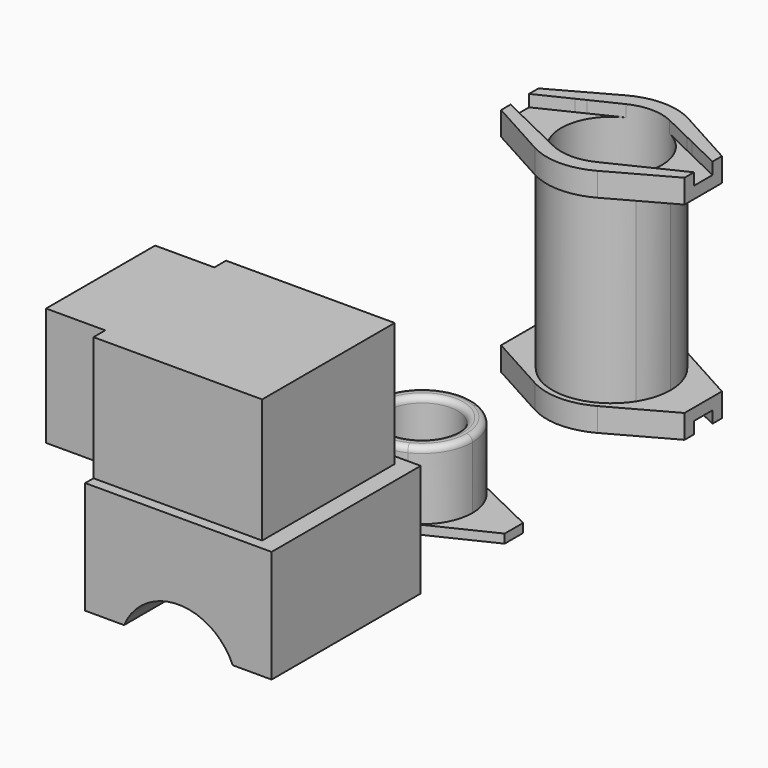
from build123d import *

# Parameters (mm, degrees)
F1_DEPTH  = 1.905
F0_R      = 7.5565
F2_DEPTH  = 16.51
F3_R      = 1.27
F5_DEPTH  = 49.53
F6_DEPTH  = 44.45
F7_DEPTH  = 5.08
F8_DEPTH  = 49.53
F9_DEPTH  = 46.99
F10_DEPTH = 44.45
F11_DEPTH = 5.08
F12_DEPTH = 2.54
F13_DEPTH = 49.53
F15_DEPTH = 24.13
F16_DEPTH = 50.8
F14_W     = 12.7
F14_H     = 29.2608
F17_DEPTH = 50.8
F18_DEPTH = 15.875
F19_DEPTH = 25.4
F21_DEPTH = 5.08
F22_DEPTH = 40.005


# Not quite as in the source:
# - after a boolean that leaves OpenCascade's solid faulty, fix() repairs it


with BuildPart() as f1:
    # F0 (on Top) → F1 (new body)
    with BuildSketch(Plane.XY):
        with BuildLine():
            ThreePointArc((-4.6970553339, -9.7195522628), (-10.795, -1.92e-08), (-4.6970553686, 9.7195522461))
            Line((-4.6970553686, 9.7195522461), (-19.685, 2.4765))
            Line((-19.685, 2.4765), (-19.685, -2.4765))
            Line((-19.685, -2.4765), (-4.6970553339, -9.7195522628))
        make_face()
    extrude(amount=F1_DEPTH)



with BuildPart() as f1b:
    # F0 (on Top) → F1, piece 2 (new body)
    with BuildSketch(Plane.XY):
        with BuildLine():
            ThreePointArc((4.6970552092, 9.7195523231), (9.1443079559, 5.7370425315), (10.795, 0))
            ThreePointArc((10.795, 0), (9.1443079608, -5.7370425236), (4.697055226, -9.719552315))
            Line((4.697055226, -9.719552315), (19.685, -2.4765))
            Line((19.685, -2.4765), (19.685, 2.4765))
            Line((19.685, 2.4765), (4.6970552092, 9.7195523231))
        make_face()
    extrude(amount=F1_DEPTH)


with BuildPart() as f1_1:
    add(f1.part)

    add(f1b.part)  # F2 merges F1b
    # F0 (on Top) → F2 (join)
    with BuildSketch(Plane.XY):
        with BuildLine():
            ThreePointArc((4.697055226, -9.719552315), (9.1443079608, -5.7370425236), (10.795, 0))
            ThreePointArc((10.795, 0), (9.1443079559, 5.7370425315), (4.6970552092, 9.7195523231))
            ThreePointArc((4.6970552092, 9.7195523231), (-8.85e-08, 10.795), (-4.6970553686, 9.7195522461))
            ThreePointArc((-4.6970553686, 9.7195522461), (-10.795, -1.92e-08), (-4.6970553339, -9.7195522628))
            ThreePointArc((-4.6970553339, -9.7195522628), (-5.99e-08, -10.795), (4.697055226, -9.719552315))
        make_face()
        Circle(F0_R, mode=Mode.SUBTRACT)
    extrude(amount=F2_DEPTH)

    # F3
    f3_edges = [f1_1.edges().sort_by_distance(p)[0] for p in [
        (-7.5565, 0, 16.51),
        (-4.697055, -9.719552, 16.51),
    ]]
    fillet(f3_edges, radius=F3_R)


with BuildPart() as f5:
    # F4 (on Top) → F5 (new body)
    with BuildSketch(Plane.XY):
        with BuildLine():
            ThreePointArc((-6.7218508036, 38.6259512066), (-10.1522301266, 41.2961604755), (-12.5905662524, 44.8950543022))
            Line((-12.5905662524, 44.8950543022), (-19.685, 48.3235))
            Line((-19.685, 48.3235), (-19.685, 45.7835))
            Line((-19.685, 45.7835), (-6.7218508036, 38.6259512066))
        make_face()
        with BuildLine():
            Line((19.685, 48.3235), (12.5905662524, 44.8950543022))
            ThreePointArc((12.5905662524, 44.8950543022), (10.1522300664, 41.2961604112), (6.7218506494, 38.6259511215))
            Line((6.7218506494, 38.6259511215), (19.685, 45.7835))
            Line((19.685, 45.7835), (19.685, 48.3235))
        make_face()
        with BuildLine():
            ThreePointArc((6.7218505572, 62.9740489294), (10.1522300304, 60.3038396273), (12.5905662524, 56.7049456978))
            Line((12.5905662524, 56.7049456978), (19.685, 53.2765))
            Line((19.685, 53.2765), (19.685, 55.8165))
            Line((19.685, 55.8165), (6.7218505572, 62.9740489294))
        make_face()
        with BuildLine():
            Line((-19.685, 53.2765), (-12.5905662524, 56.7049456978))
            ThreePointArc((-12.5905662524, 56.7049456978), (-10.1522299741, 60.3038396874), (-6.721850413, 62.9740490091))
            Line((-6.721850413, 62.9740490091), (-19.685, 55.8165))
            Line((-19.685, 55.8165), (-19.685, 53.2765))
        make_face()
        with BuildLine():
            ThreePointArc((-12.5905662524, 44.8950543022), (-13.9065, 50.8), (-12.5905662524, 56.7049456978))
            Line((-12.5905662524, 56.7049456978), (-19.685, 53.2765))
            Line((-19.685, 53.2765), (-19.685, 48.3235))
            Line((-19.685, 48.3235), (-12.5905662524, 44.8950543022))
        make_face()
        with BuildLine():
            Line((19.685, 53.2765), (12.5905662524, 56.7049456978))
            ThreePointArc((12.5905662524, 56.7049456978), (13.5735303411, 53.8248993918), (13.9065, 50.8))
            ThreePointArc((13.9065, 50.8), (13.5735303411, 47.7751006082), (12.5905662524, 44.8950543022))
            Line((12.5905662524, 44.8950543022), (19.685, 48.3235))
            Line((19.685, 48.3235), (19.685, 53.2765))
        make_face()
        with BuildLine():
            ThreePointArc((-10.7206935622, 43.9914223552), (-12.7, 50.8), (-10.7206935622, 57.6085776448))
            Line((-10.7206935622, 57.6085776448), (-12.5905662524, 56.7049456978))
            ThreePointArc((-12.5905662524, 56.7049456978), (-13.9065, 50.8), (-12.5905662524, 44.8950543022))
            Line((-12.5905662524, 44.8950543022), (-10.7206935622, 43.9914223552))
        make_face()
        with BuildLine():
            ThreePointArc((-10.7206935622, 57.6085776448), (0, 63.5), (10.7206935622, 57.6085776448))
            Line((10.7206935622, 57.6085776448), (12.5905662524, 56.7049456978))
            ThreePointArc((12.5905662524, 56.7049456978), (10.1522300304, 60.3038396273), (6.7218505572, 62.9740489294))
            ThreePointArc((6.7218505572, 62.9740489294), (8.24e-08, 64.7065), (-6.721850413, 62.9740490091))
            ThreePointArc((-6.721850413, 62.9740490091), (-10.1522299741, 60.3038396874), (-12.5905662524, 56.7049456978))
            Line((-12.5905662524, 56.7049456978), (-10.7206935622, 57.6085776448))
        make_face()
        with BuildLine():
            ThreePointArc((-4.6970550571, 41.0804476034), (-10.795, 50.7999998253), (-4.6970553717, 60.5195522446))
            Line((-4.6970553717, 60.5195522446), (-10.7206935622, 57.6085776448))
            ThreePointArc((-10.7206935622, 57.6085776448), (-12.7, 50.8), (-10.7206935622, 43.9914223552))
            Line((-10.7206935622, 43.9914223552), (-4.6970550571, 41.0804476034))
        make_face()
        with BuildLine():
            Line((0, 62.7894443677), (4.697055398, 60.5195522319))
            Line((4.697055398, 60.5195522319), (10.7206935622, 57.6085776448))
            ThreePointArc((10.7206935622, 57.6085776448), (0, 63.5), (-10.7206935622, 57.6085776448))
            Line((-10.7206935622, 57.6085776448), (-4.6970553717, 60.5195522446))
            Line((-4.6970553717, 60.5195522446), (0, 62.7894443677))
        make_face()
        with BuildLine():
            ThreePointArc((-4.6970553717, 60.5195522446), (1.46e-08, 61.595), (4.697055398, 60.5195522319))
            Line((4.697055398, 60.5195522319), (0, 62.7894443677))
            Line((0, 62.7894443677), (-4.6970553717, 60.5195522446))
        make_face()
        with BuildLine():
            ThreePointArc((4.6970554112, 41.0804477745), (9.1443080155, 45.0629575635), (10.795, 50.8))
            ThreePointArc((10.795, 50.8), (9.1443080116, 56.5370424427), (4.697055398, 60.5195522319))
            ThreePointArc((4.697055398, 60.5195522319), (1.46e-08, 61.595), (-4.6970553717, 60.5195522446))
            ThreePointArc((-4.6970553717, 60.5195522446), (-10.795, 50.7999998253), (-4.6970550571, 41.0804476034))
            ThreePointArc((-4.6970550571, 41.0804476034), (1.966e-07, 40.005), (4.6970554112, 41.0804477745))
        make_face()
        with BuildLine():
            Line((0, 38.8105556323), (4.6970554112, 41.0804477745))
            ThreePointArc((4.6970554112, 41.0804477745), (1.966e-07, 40.005), (-4.6970550571, 41.0804476034))
            Line((-4.6970550571, 41.0804476034), (0, 38.8105556323))
        make_face()
        with BuildLine():
            Line((10.7206935622, 43.9914223552), (4.6970554112, 41.0804477745))
            Line((4.6970554112, 41.0804477745), (0, 38.8105556323))
            Line((0, 38.8105556323), (-4.6970550571, 41.0804476034))
            Line((-4.6970550571, 41.0804476034), (-10.7206935622, 43.9914223552))
            ThreePointArc((-10.7206935622, 43.9914223552), (0, 38.1), (10.7206935622, 43.9914223552))
        make_face()
        with BuildLine():
            Line((12.5905662524, 44.8950543022), (10.7206935622, 43.9914223552))
            ThreePointArc((10.7206935622, 43.9914223552), (0, 38.1), (-10.7206935622, 43.9914223552))
            Line((-10.7206935622, 43.9914223552), (-12.5905662524, 44.8950543022))
            ThreePointArc((-12.5905662524, 44.8950543022), (-10.1522301266, 41.2961604755), (-6.7218508036, 38.6259512066))
            ThreePointArc((-6.7218508036, 38.6259512066), (-8.81e-08, 36.8935), (6.7218506494, 38.6259511215))
            ThreePointArc((6.7218506494, 38.6259511215), (10.1522300664, 41.2961604112), (12.5905662524, 44.8950543022))
        make_face()
        with BuildLine():
            ThreePointArc((4.697055398, 60.5195522319), (9.1443080116, 56.5370424427), (10.795, 50.8))
            ThreePointArc((10.795, 50.8), (9.1443080155, 45.0629575635), (4.6970554112, 41.0804477745))
            Line((4.6970554112, 41.0804477745), (10.7206935622, 43.9914223552))
            ThreePointArc((10.7206935622, 43.9914223552), (12.1951385445, 47.2547784442), (12.7, 50.8))
            ThreePointArc((12.7, 50.8), (12.1951385445, 54.3452215558), (10.7206935622, 57.6085776448))
            Line((10.7206935622, 57.6085776448), (4.697055398, 60.5195522319))
        make_face()
        with BuildLine():
            Line((12.5905662524, 56.7049456978), (10.7206935622, 57.6085776448))
            ThreePointArc((10.7206935622, 57.6085776448), (12.1951385445, 54.3452215558), (12.7, 50.8))
            ThreePointArc((12.7, 50.8), (12.1951385445, 47.2547784442), (10.7206935622, 43.9914223552))
            Line((10.7206935622, 43.9914223552), (12.5905662524, 44.8950543022))
            ThreePointArc((12.5905662524, 44.8950543022), (13.5735303411, 47.7751006082), (13.9065, 50.8))
            ThreePointArc((13.9065, 50.8), (13.5735303411, 53.8248993918), (12.5905662524, 56.7049456978))
        make_face()
    extrude(amount=F5_DEPTH)

    # F4 (on Top) → F6 (cut)
    with BuildSketch(Plane.XY):
        with BuildLine():
            ThreePointArc((-6.7218508036, 38.6259512066), (-10.1522301266, 41.2961604755), (-12.5905662524, 44.8950543022))
            Line((-12.5905662524, 44.8950543022), (-19.685, 48.3235))
            Line((-19.685, 48.3235), (-19.685, 45.7835))
            Line((-19.685, 45.7835), (-6.7218508036, 38.6259512066))
        make_face()
        with BuildLine():
            ThreePointArc((-12.5905662524, 44.8950543022), (-13.9065, 50.8), (-12.5905662524, 56.7049456978))
            Line((-12.5905662524, 56.7049456978), (-19.685, 53.2765))
            Line((-19.685, 53.2765), (-19.685, 48.3235))
            Line((-19.685, 48.3235), (-12.5905662524, 44.8950543022))
        make_face()
        with BuildLine():
            Line((-19.685, 53.2765), (-12.5905662524, 56.7049456978))
            ThreePointArc((-12.5905662524, 56.7049456978), (-10.1522299741, 60.3038396874), (-6.721850413, 62.9740490091))
            Line((-6.721850413, 62.9740490091), (-19.685, 55.8165))
            Line((-19.685, 55.8165), (-19.685, 53.2765))
        make_face()
        with BuildLine():
            ThreePointArc((6.7218505572, 62.9740489294), (10.1522300304, 60.3038396273), (12.5905662524, 56.7049456978))
            Line((12.5905662524, 56.7049456978), (19.685, 53.2765))
            Line((19.685, 53.2765), (19.685, 55.8165))
            Line((19.685, 55.8165), (6.7218505572, 62.9740489294))
        make_face()
        with BuildLine():
            Line((19.685, 53.2765), (12.5905662524, 56.7049456978))
            ThreePointArc((12.5905662524, 56.7049456978), (13.5735303411, 53.8248993918), (13.9065, 50.8))
            ThreePointArc((13.9065, 50.8), (13.5735303411, 47.7751006082), (12.5905662524, 44.8950543022))
            Line((12.5905662524, 44.8950543022), (19.685, 48.3235))
            Line((19.685, 48.3235), (19.685, 53.2765))
        make_face()
        with BuildLine():
            Line((19.685, 48.3235), (12.5905662524, 44.8950543022))
            ThreePointArc((12.5905662524, 44.8950543022), (10.1522300664, 41.2961604112), (6.7218506494, 38.6259511215))
            Line((6.7218506494, 38.6259511215), (19.685, 45.7835))
            Line((19.685, 45.7835), (19.685, 48.3235))
        make_face()
        with BuildLine():
            Line((12.5905662524, 44.8950543022), (10.7206935622, 43.9914223552))
            ThreePointArc((10.7206935622, 43.9914223552), (0, 38.1), (-10.7206935622, 43.9914223552))
            Line((-10.7206935622, 43.9914223552), (-12.5905662524, 44.8950543022))
            ThreePointArc((-12.5905662524, 44.8950543022), (-10.1522301266, 41.2961604755), (-6.7218508036, 38.6259512066))
            ThreePointArc((-6.7218508036, 38.6259512066), (-8.81e-08, 36.8935), (6.7218506494, 38.6259511215))
            ThreePointArc((6.7218506494, 38.6259511215), (10.1522300664, 41.2961604112), (12.5905662524, 44.8950543022))
        make_face()
        with BuildLine():
            ThreePointArc((-10.7206935622, 57.6085776448), (0, 63.5), (10.7206935622, 57.6085776448))
            Line((10.7206935622, 57.6085776448), (12.5905662524, 56.7049456978))
            ThreePointArc((12.5905662524, 56.7049456978), (10.1522300304, 60.3038396273), (6.7218505572, 62.9740489294))
            ThreePointArc((6.7218505572, 62.9740489294), (8.24e-08, 64.7065), (-6.721850413, 62.9740490091))
            ThreePointArc((-6.721850413, 62.9740490091), (-10.1522299741, 60.3038396874), (-12.5905662524, 56.7049456978))
            Line((-12.5905662524, 56.7049456978), (-10.7206935622, 57.6085776448))
        make_face()
        with BuildLine():
            Line((12.5905662524, 56.7049456978), (10.7206935622, 57.6085776448))
            ThreePointArc((10.7206935622, 57.6085776448), (12.1951385445, 54.3452215558), (12.7, 50.8))
            ThreePointArc((12.7, 50.8), (12.1951385445, 47.2547784442), (10.7206935622, 43.9914223552))
            Line((10.7206935622, 43.9914223552), (12.5905662524, 44.8950543022))
            ThreePointArc((12.5905662524, 44.8950543022), (13.5735303411, 47.7751006082), (13.9065, 50.8))
            ThreePointArc((13.9065, 50.8), (13.5735303411, 53.8248993918), (12.5905662524, 56.7049456978))
        make_face()
        with BuildLine():
            ThreePointArc((-10.7206935622, 43.9914223552), (-12.7, 50.8), (-10.7206935622, 57.6085776448))
            Line((-10.7206935622, 57.6085776448), (-12.5905662524, 56.7049456978))
            ThreePointArc((-12.5905662524, 56.7049456978), (-13.9065, 50.8), (-12.5905662524, 44.8950543022))
            Line((-12.5905662524, 44.8950543022), (-10.7206935622, 43.9914223552))
        make_face()
    extrude(amount=F6_DEPTH, mode=Mode.SUBTRACT)

    # F4 (on Top) → F7 (join)
    with BuildSketch(Plane.XY):
        with BuildLine():
            ThreePointArc((-6.7218508036, 38.6259512066), (-10.1522301266, 41.2961604755), (-12.5905662524, 44.8950543022))
            Line((-12.5905662524, 44.8950543022), (-19.685, 48.3235))
            Line((-19.685, 48.3235), (-19.685, 45.7835))
            Line((-19.685, 45.7835), (-6.7218508036, 38.6259512066))
        make_face()
        with BuildLine():
            Line((12.5905662524, 44.8950543022), (10.7206935622, 43.9914223552))
            ThreePointArc((10.7206935622, 43.9914223552), (0, 38.1), (-10.7206935622, 43.9914223552))
            Line((-10.7206935622, 43.9914223552), (-12.5905662524, 44.8950543022))
            ThreePointArc((-12.5905662524, 44.8950543022), (-10.1522301266, 41.2961604755), (-6.7218508036, 38.6259512066))
            ThreePointArc((-6.7218508036, 38.6259512066), (-8.81e-08, 36.8935), (6.7218506494, 38.6259511215))
            ThreePointArc((6.7218506494, 38.6259511215), (10.1522300664, 41.2961604112), (12.5905662524, 44.8950543022))
        make_face()
        with BuildLine():
            Line((10.7206935622, 43.9914223552), (4.6970554112, 41.0804477745))
            Line((4.6970554112, 41.0804477745), (0, 38.8105556323))
            Line((0, 38.8105556323), (-4.6970550571, 41.0804476034))
            Line((-4.6970550571, 41.0804476034), (-10.7206935622, 43.9914223552))
            ThreePointArc((-10.7206935622, 43.9914223552), (0, 38.1), (10.7206935622, 43.9914223552))
        make_face()
        with BuildLine():
            ThreePointArc((-4.6970550571, 41.0804476034), (-10.795, 50.7999998253), (-4.6970553717, 60.5195522446))
            Line((-4.6970553717, 60.5195522446), (-10.7206935622, 57.6085776448))
            ThreePointArc((-10.7206935622, 57.6085776448), (-12.7, 50.8), (-10.7206935622, 43.9914223552))
            Line((-10.7206935622, 43.9914223552), (-4.6970550571, 41.0804476034))
        make_face()
        with BuildLine():
            ThreePointArc((-10.7206935622, 43.9914223552), (-12.7, 50.8), (-10.7206935622, 57.6085776448))
            Line((-10.7206935622, 57.6085776448), (-12.5905662524, 56.7049456978))
            ThreePointArc((-12.5905662524, 56.7049456978), (-13.9065, 50.8), (-12.5905662524, 44.8950543022))
            Line((-12.5905662524, 44.8950543022), (-10.7206935622, 43.9914223552))
        make_face()
        with BuildLine():
            ThreePointArc((-12.5905662524, 44.8950543022), (-13.9065, 50.8), (-12.5905662524, 56.7049456978))
            Line((-12.5905662524, 56.7049456978), (-19.685, 53.2765))
            Line((-19.685, 53.2765), (-19.685, 48.3235))
            Line((-19.685, 48.3235), (-12.5905662524, 44.8950543022))
        make_face()
        with BuildLine():
            Line((-19.685, 53.2765), (-12.5905662524, 56.7049456978))
            ThreePointArc((-12.5905662524, 56.7049456978), (-10.1522299741, 60.3038396874), (-6.721850413, 62.9740490091))
            Line((-6.721850413, 62.9740490091), (-19.685, 55.8165))
            Line((-19.685, 55.8165), (-19.685, 53.2765))
        make_face()
        with BuildLine():
            Line((0, 62.7894443677), (4.697055398, 60.5195522319))
            Line((4.697055398, 60.5195522319), (10.7206935622, 57.6085776448))
            ThreePointArc((10.7206935622, 57.6085776448), (0, 63.5), (-10.7206935622, 57.6085776448))
            Line((-10.7206935622, 57.6085776448), (-4.6970553717, 60.5195522446))
            Line((-4.6970553717, 60.5195522446), (0, 62.7894443677))
        make_face()
        with BuildLine():
            ThreePointArc((-10.7206935622, 57.6085776448), (0, 63.5), (10.7206935622, 57.6085776448))
            Line((10.7206935622, 57.6085776448), (12.5905662524, 56.7049456978))
            ThreePointArc((12.5905662524, 56.7049456978), (10.1522300304, 60.3038396273), (6.7218505572, 62.9740489294))
            ThreePointArc((6.7218505572, 62.9740489294), (8.24e-08, 64.7065), (-6.721850413, 62.9740490091))
            ThreePointArc((-6.721850413, 62.9740490091), (-10.1522299741, 60.3038396874), (-12.5905662524, 56.7049456978))
            Line((-12.5905662524, 56.7049456978), (-10.7206935622, 57.6085776448))
        make_face()
        with BuildLine():
            ThreePointArc((-4.6970553717, 60.5195522446), (1.46e-08, 61.595), (4.697055398, 60.5195522319))
            Line((4.697055398, 60.5195522319), (0, 62.7894443677))
            Line((0, 62.7894443677), (-4.6970553717, 60.5195522446))
        make_face()
        with BuildLine():
            ThreePointArc((4.6970554112, 41.0804477745), (9.1443080155, 45.0629575635), (10.795, 50.8))
            ThreePointArc((10.795, 50.8), (9.1443080116, 56.5370424427), (4.697055398, 60.5195522319))
            ThreePointArc((4.697055398, 60.5195522319), (1.46e-08, 61.595), (-4.6970553717, 60.5195522446))
            ThreePointArc((-4.6970553717, 60.5195522446), (-10.795, 50.7999998253), (-4.6970550571, 41.0804476034))
            ThreePointArc((-4.6970550571, 41.0804476034), (1.966e-07, 40.005), (4.6970554112, 41.0804477745))
        make_face()
        with BuildLine():
            ThreePointArc((4.697055398, 60.5195522319), (9.1443080116, 56.5370424427), (10.795, 50.8))
            ThreePointArc((10.795, 50.8), (9.1443080155, 45.0629575635), (4.6970554112, 41.0804477745))
            Line((4.6970554112, 41.0804477745), (10.7206935622, 43.9914223552))
            ThreePointArc((10.7206935622, 43.9914223552), (12.1951385445, 47.2547784442), (12.7, 50.8))
            ThreePointArc((12.7, 50.8), (12.1951385445, 54.3452215558), (10.7206935622, 57.6085776448))
            Line((10.7206935622, 57.6085776448), (4.697055398, 60.5195522319))
        make_face()
        with BuildLine():
            Line((12.5905662524, 56.7049456978), (10.7206935622, 57.6085776448))
            ThreePointArc((10.7206935622, 57.6085776448), (12.1951385445, 54.3452215558), (12.7, 50.8))
            ThreePointArc((12.7, 50.8), (12.1951385445, 47.2547784442), (10.7206935622, 43.9914223552))
            Line((10.7206935622, 43.9914223552), (12.5905662524, 44.8950543022))
            ThreePointArc((12.5905662524, 44.8950543022), (13.5735303411, 47.7751006082), (13.9065, 50.8))
            ThreePointArc((13.9065, 50.8), (13.5735303411, 53.8248993918), (12.5905662524, 56.7049456978))
        make_face()
        with BuildLine():
            Line((19.685, 53.2765), (12.5905662524, 56.7049456978))
            ThreePointArc((12.5905662524, 56.7049456978), (13.5735303411, 53.8248993918), (13.9065, 50.8))
            ThreePointArc((13.9065, 50.8), (13.5735303411, 47.7751006082), (12.5905662524, 44.8950543022))
            Line((12.5905662524, 44.8950543022), (19.685, 48.3235))
            Line((19.685, 48.3235), (19.685, 53.2765))
        make_face()
        with BuildLine():
            ThreePointArc((6.7218505572, 62.9740489294), (10.1522300304, 60.3038396273), (12.5905662524, 56.7049456978))
            Line((12.5905662524, 56.7049456978), (19.685, 53.2765))
            Line((19.685, 53.2765), (19.685, 55.8165))
            Line((19.685, 55.8165), (6.7218505572, 62.9740489294))
        make_face()
        with BuildLine():
            Line((19.685, 48.3235), (12.5905662524, 44.8950543022))
            ThreePointArc((12.5905662524, 44.8950543022), (10.1522300664, 41.2961604112), (6.7218506494, 38.6259511215))
            Line((6.7218506494, 38.6259511215), (19.685, 45.7835))
            Line((19.685, 45.7835), (19.685, 48.3235))
        make_face()
        with BuildLine():
            Line((0, 38.8105556323), (4.6970554112, 41.0804477745))
            ThreePointArc((4.6970554112, 41.0804477745), (1.966e-07, 40.005), (-4.6970550571, 41.0804476034))
            Line((-4.6970550571, 41.0804476034), (0, 38.8105556323))
        make_face()
    extrude(amount=F7_DEPTH)

    # F4 (on Top) → F8 (cut)
    with BuildSketch(Plane.XY):
        with BuildLine():
            ThreePointArc((-12.5905662524, 44.8950543022), (-13.9065, 50.8), (-12.5905662524, 56.7049456978))
            Line((-12.5905662524, 56.7049456978), (-19.685, 53.2765))
            Line((-19.685, 53.2765), (-19.685, 48.3235))
            Line((-19.685, 48.3235), (-12.5905662524, 44.8950543022))
        make_face()
        with BuildLine():
            ThreePointArc((-10.7206935622, 43.9914223552), (-12.7, 50.8), (-10.7206935622, 57.6085776448))
            Line((-10.7206935622, 57.6085776448), (-12.5905662524, 56.7049456978))
            ThreePointArc((-12.5905662524, 56.7049456978), (-13.9065, 50.8), (-12.5905662524, 44.8950543022))
            Line((-12.5905662524, 44.8950543022), (-10.7206935622, 43.9914223552))
        make_face()
        with BuildLine():
            ThreePointArc((-4.6970550571, 41.0804476034), (-10.795, 50.7999998253), (-4.6970553717, 60.5195522446))
            Line((-4.6970553717, 60.5195522446), (-10.7206935622, 57.6085776448))
            ThreePointArc((-10.7206935622, 57.6085776448), (-12.7, 50.8), (-10.7206935622, 43.9914223552))
            Line((-10.7206935622, 43.9914223552), (-4.6970550571, 41.0804476034))
        make_face()
        with BuildLine():
            ThreePointArc((4.6970554112, 41.0804477745), (9.1443080155, 45.0629575635), (10.795, 50.8))
            ThreePointArc((10.795, 50.8), (9.1443080116, 56.5370424427), (4.697055398, 60.5195522319))
            ThreePointArc((4.697055398, 60.5195522319), (1.46e-08, 61.595), (-4.6970553717, 60.5195522446))
            ThreePointArc((-4.6970553717, 60.5195522446), (-10.795, 50.7999998253), (-4.6970550571, 41.0804476034))
            ThreePointArc((-4.6970550571, 41.0804476034), (1.966e-07, 40.005), (4.6970554112, 41.0804477745))
        make_face()
        with BuildLine():
            ThreePointArc((4.697055398, 60.5195522319), (9.1443080116, 56.5370424427), (10.795, 50.8))
            ThreePointArc((10.795, 50.8), (9.1443080155, 45.0629575635), (4.6970554112, 41.0804477745))
            Line((4.6970554112, 41.0804477745), (10.7206935622, 43.9914223552))
            ThreePointArc((10.7206935622, 43.9914223552), (12.1951385445, 47.2547784442), (12.7, 50.8))
            ThreePointArc((12.7, 50.8), (12.1951385445, 54.3452215558), (10.7206935622, 57.6085776448))
            Line((10.7206935622, 57.6085776448), (4.697055398, 60.5195522319))
        make_face()
        with BuildLine():
            Line((12.5905662524, 56.7049456978), (10.7206935622, 57.6085776448))
            ThreePointArc((10.7206935622, 57.6085776448), (12.1951385445, 54.3452215558), (12.7, 50.8))
            ThreePointArc((12.7, 50.8), (12.1951385445, 47.2547784442), (10.7206935622, 43.9914223552))
            Line((10.7206935622, 43.9914223552), (12.5905662524, 44.8950543022))
            ThreePointArc((12.5905662524, 44.8950543022), (13.5735303411, 47.7751006082), (13.9065, 50.8))
            ThreePointArc((13.9065, 50.8), (13.5735303411, 53.8248993918), (12.5905662524, 56.7049456978))
        make_face()
        with BuildLine():
            Line((19.685, 53.2765), (12.5905662524, 56.7049456978))
            ThreePointArc((12.5905662524, 56.7049456978), (13.5735303411, 53.8248993918), (13.9065, 50.8))
            ThreePointArc((13.9065, 50.8), (13.5735303411, 47.7751006082), (12.5905662524, 44.8950543022))
            Line((12.5905662524, 44.8950543022), (19.685, 48.3235))
            Line((19.685, 48.3235), (19.685, 53.2765))
        make_face()
    extrude(amount=F8_DEPTH, mode=Mode.SUBTRACT)

    # F4 (on Top) → F9 (join)
    with BuildSketch(Plane.XY):
        with BuildLine():
            ThreePointArc((-12.5905662524, 44.8950543022), (-13.9065, 50.8), (-12.5905662524, 56.7049456978))
            Line((-12.5905662524, 56.7049456978), (-19.685, 53.2765))
            Line((-19.685, 53.2765), (-19.685, 48.3235))
            Line((-19.685, 48.3235), (-12.5905662524, 44.8950543022))
        make_face()
        with BuildLine():
            ThreePointArc((-10.7206935622, 43.9914223552), (-12.7, 50.8), (-10.7206935622, 57.6085776448))
            Line((-10.7206935622, 57.6085776448), (-12.5905662524, 56.7049456978))
            ThreePointArc((-12.5905662524, 56.7049456978), (-13.9065, 50.8), (-12.5905662524, 44.8950543022))
            Line((-12.5905662524, 44.8950543022), (-10.7206935622, 43.9914223552))
        make_face()
        with BuildLine():
            ThreePointArc((-4.6970550571, 41.0804476034), (-10.795, 50.7999998253), (-4.6970553717, 60.5195522446))
            Line((-4.6970553717, 60.5195522446), (-10.7206935622, 57.6085776448))
            ThreePointArc((-10.7206935622, 57.6085776448), (-12.7, 50.8), (-10.7206935622, 43.9914223552))
            Line((-10.7206935622, 43.9914223552), (-4.6970550571, 41.0804476034))
        make_face()
        with BuildLine():
            ThreePointArc((4.6970554112, 41.0804477745), (9.1443080155, 45.0629575635), (10.795, 50.8))
            ThreePointArc((10.795, 50.8), (9.1443080116, 56.5370424427), (4.697055398, 60.5195522319))
            ThreePointArc((4.697055398, 60.5195522319), (1.46e-08, 61.595), (-4.6970553717, 60.5195522446))
            ThreePointArc((-4.6970553717, 60.5195522446), (-10.795, 50.7999998253), (-4.6970550571, 41.0804476034))
            ThreePointArc((-4.6970550571, 41.0804476034), (1.966e-07, 40.005), (4.6970554112, 41.0804477745))
        make_face()
        with BuildLine():
            ThreePointArc((4.697055398, 60.5195522319), (9.1443080116, 56.5370424427), (10.795, 50.8))
            ThreePointArc((10.795, 50.8), (9.1443080155, 45.0629575635), (4.6970554112, 41.0804477745))
            Line((4.6970554112, 41.0804477745), (10.7206935622, 43.9914223552))
            ThreePointArc((10.7206935622, 43.9914223552), (12.1951385445, 47.2547784442), (12.7, 50.8))
            ThreePointArc((12.7, 50.8), (12.1951385445, 54.3452215558), (10.7206935622, 57.6085776448))
            Line((10.7206935622, 57.6085776448), (4.697055398, 60.5195522319))
        make_face()
        with BuildLine():
            Line((12.5905662524, 56.7049456978), (10.7206935622, 57.6085776448))
            ThreePointArc((10.7206935622, 57.6085776448), (12.1951385445, 54.3452215558), (12.7, 50.8))
            ThreePointArc((12.7, 50.8), (12.1951385445, 47.2547784442), (10.7206935622, 43.9914223552))
            Line((10.7206935622, 43.9914223552), (12.5905662524, 44.8950543022))
            ThreePointArc((12.5905662524, 44.8950543022), (13.5735303411, 47.7751006082), (13.9065, 50.8))
            ThreePointArc((13.9065, 50.8), (13.5735303411, 53.8248993918), (12.5905662524, 56.7049456978))
        make_face()
        with BuildLine():
            Line((19.685, 53.2765), (12.5905662524, 56.7049456978))
            ThreePointArc((12.5905662524, 56.7049456978), (13.5735303411, 53.8248993918), (13.9065, 50.8))
            ThreePointArc((13.9065, 50.8), (13.5735303411, 47.7751006082), (12.5905662524, 44.8950543022))
            Line((12.5905662524, 44.8950543022), (19.685, 48.3235))
            Line((19.685, 48.3235), (19.685, 53.2765))
        make_face()
    extrude(amount=F9_DEPTH)

    # F4 (on Top) → F10 (cut)
    with BuildSketch(Plane.XY):
        with BuildLine():
            Line((19.685, 53.2765), (12.5905662524, 56.7049456978))
            ThreePointArc((12.5905662524, 56.7049456978), (13.5735303411, 53.8248993918), (13.9065, 50.8))
            ThreePointArc((13.9065, 50.8), (13.5735303411, 47.7751006082), (12.5905662524, 44.8950543022))
            Line((12.5905662524, 44.8950543022), (19.685, 48.3235))
            Line((19.685, 48.3235), (19.685, 53.2765))
        make_face()
        with BuildLine():
            Line((12.5905662524, 56.7049456978), (10.7206935622, 57.6085776448))
            ThreePointArc((10.7206935622, 57.6085776448), (12.1951385445, 54.3452215558), (12.7, 50.8))
            ThreePointArc((12.7, 50.8), (12.1951385445, 47.2547784442), (10.7206935622, 43.9914223552))
            Line((10.7206935622, 43.9914223552), (12.5905662524, 44.8950543022))
            ThreePointArc((12.5905662524, 44.8950543022), (13.5735303411, 47.7751006082), (13.9065, 50.8))
            ThreePointArc((13.9065, 50.8), (13.5735303411, 53.8248993918), (12.5905662524, 56.7049456978))
        make_face()
        with BuildLine():
            ThreePointArc((-12.5905662524, 44.8950543022), (-13.9065, 50.8), (-12.5905662524, 56.7049456978))
            Line((-12.5905662524, 56.7049456978), (-19.685, 53.2765))
            Line((-19.685, 53.2765), (-19.685, 48.3235))
            Line((-19.685, 48.3235), (-12.5905662524, 44.8950543022))
        make_face()
        with BuildLine():
            ThreePointArc((-10.7206935622, 43.9914223552), (-12.7, 50.8), (-10.7206935622, 57.6085776448))
            Line((-10.7206935622, 57.6085776448), (-12.5905662524, 56.7049456978))
            ThreePointArc((-12.5905662524, 56.7049456978), (-13.9065, 50.8), (-12.5905662524, 44.8950543022))
            Line((-12.5905662524, 44.8950543022), (-10.7206935622, 43.9914223552))
        make_face()
    extrude(amount=F10_DEPTH, mode=Mode.SUBTRACT)

    # F4 (on Top) → F11 (join)
    with BuildSketch(Plane.XY):
        with BuildLine():
            Line((19.685, 53.2765), (12.5905662524, 56.7049456978))
            ThreePointArc((12.5905662524, 56.7049456978), (13.5735303411, 53.8248993918), (13.9065, 50.8))
            ThreePointArc((13.9065, 50.8), (13.5735303411, 47.7751006082), (12.5905662524, 44.8950543022))
            Line((12.5905662524, 44.8950543022), (19.685, 48.3235))
            Line((19.685, 48.3235), (19.685, 53.2765))
        make_face()
        with BuildLine():
            Line((12.5905662524, 56.7049456978), (10.7206935622, 57.6085776448))
            ThreePointArc((10.7206935622, 57.6085776448), (12.1951385445, 54.3452215558), (12.7, 50.8))
            ThreePointArc((12.7, 50.8), (12.1951385445, 47.2547784442), (10.7206935622, 43.9914223552))
            Line((10.7206935622, 43.9914223552), (12.5905662524, 44.8950543022))
            ThreePointArc((12.5905662524, 44.8950543022), (13.5735303411, 47.7751006082), (13.9065, 50.8))
            ThreePointArc((13.9065, 50.8), (13.5735303411, 53.8248993918), (12.5905662524, 56.7049456978))
        make_face()
        with BuildLine():
            ThreePointArc((-10.7206935622, 43.9914223552), (-12.7, 50.8), (-10.7206935622, 57.6085776448))
            Line((-10.7206935622, 57.6085776448), (-12.5905662524, 56.7049456978))
            ThreePointArc((-12.5905662524, 56.7049456978), (-13.9065, 50.8), (-12.5905662524, 44.8950543022))
            Line((-12.5905662524, 44.8950543022), (-10.7206935622, 43.9914223552))
        make_face()
        with BuildLine():
            ThreePointArc((-12.5905662524, 44.8950543022), (-13.9065, 50.8), (-12.5905662524, 56.7049456978))
            Line((-12.5905662524, 56.7049456978), (-19.685, 53.2765))
            Line((-19.685, 53.2765), (-19.685, 48.3235))
            Line((-19.685, 48.3235), (-12.5905662524, 44.8950543022))
        make_face()
    extrude(amount=F11_DEPTH)

    # F4 (on Top) → F12 (cut)
    with BuildSketch(Plane.XY):
        with BuildLine():
            ThreePointArc((-12.5905662524, 44.8950543022), (-13.9065, 50.8), (-12.5905662524, 56.7049456978))
            Line((-12.5905662524, 56.7049456978), (-19.685, 53.2765))
            Line((-19.685, 53.2765), (-19.685, 48.3235))
            Line((-19.685, 48.3235), (-12.5905662524, 44.8950543022))
        make_face()
        with BuildLine():
            ThreePointArc((-10.7206935622, 43.9914223552), (-12.7, 50.8), (-10.7206935622, 57.6085776448))
            Line((-10.7206935622, 57.6085776448), (-12.5905662524, 56.7049456978))
            ThreePointArc((-12.5905662524, 56.7049456978), (-13.9065, 50.8), (-12.5905662524, 44.8950543022))
            Line((-12.5905662524, 44.8950543022), (-10.7206935622, 43.9914223552))
        make_face()
        with BuildLine():
            ThreePointArc((-4.6970550571, 41.0804476034), (-10.795, 50.7999998253), (-4.6970553717, 60.5195522446))
            Line((-4.6970553717, 60.5195522446), (-10.7206935622, 57.6085776448))
            ThreePointArc((-10.7206935622, 57.6085776448), (-12.7, 50.8), (-10.7206935622, 43.9914223552))
            Line((-10.7206935622, 43.9914223552), (-4.6970550571, 41.0804476034))
        make_face()
        with BuildLine():
            ThreePointArc((4.6970554112, 41.0804477745), (9.1443080155, 45.0629575635), (10.795, 50.8))
            ThreePointArc((10.795, 50.8), (9.1443080116, 56.5370424427), (4.697055398, 60.5195522319))
            ThreePointArc((4.697055398, 60.5195522319), (1.46e-08, 61.595), (-4.6970553717, 60.5195522446))
            ThreePointArc((-4.6970553717, 60.5195522446), (-10.795, 50.7999998253), (-4.6970550571, 41.0804476034))
            ThreePointArc((-4.6970550571, 41.0804476034), (1.966e-07, 40.005), (4.6970554112, 41.0804477745))
        make_face()
        with BuildLine():
            ThreePointArc((4.697055398, 60.5195522319), (9.1443080116, 56.5370424427), (10.795, 50.8))
            ThreePointArc((10.795, 50.8), (9.1443080155, 45.0629575635), (4.6970554112, 41.0804477745))
            Line((4.6970554112, 41.0804477745), (10.7206935622, 43.9914223552))
            ThreePointArc((10.7206935622, 43.9914223552), (12.1951385445, 47.2547784442), (12.7, 50.8))
            ThreePointArc((12.7, 50.8), (12.1951385445, 54.3452215558), (10.7206935622, 57.6085776448))
            Line((10.7206935622, 57.6085776448), (4.697055398, 60.5195522319))
        make_face()
        with BuildLine():
            Line((12.5905662524, 56.7049456978), (10.7206935622, 57.6085776448))
            ThreePointArc((10.7206935622, 57.6085776448), (12.1951385445, 54.3452215558), (12.7, 50.8))
            ThreePointArc((12.7, 50.8), (12.1951385445, 47.2547784442), (10.7206935622, 43.9914223552))
            Line((10.7206935622, 43.9914223552), (12.5905662524, 44.8950543022))
            ThreePointArc((12.5905662524, 44.8950543022), (13.5735303411, 47.7751006082), (13.9065, 50.8))
            ThreePointArc((13.9065, 50.8), (13.5735303411, 53.8248993918), (12.5905662524, 56.7049456978))
        make_face()
        with BuildLine():
            Line((19.685, 53.2765), (12.5905662524, 56.7049456978))
            ThreePointArc((12.5905662524, 56.7049456978), (13.5735303411, 53.8248993918), (13.9065, 50.8))
            ThreePointArc((13.9065, 50.8), (13.5735303411, 47.7751006082), (12.5905662524, 44.8950543022))
            Line((12.5905662524, 44.8950543022), (19.685, 48.3235))
            Line((19.685, 48.3235), (19.685, 53.2765))
        make_face()
    extrude(amount=F12_DEPTH, mode=Mode.SUBTRACT)

    # F4 (on Top) → F13 (cut)
    with BuildSketch(Plane.XY):
        with BuildLine():
            ThreePointArc((4.6970554112, 41.0804477745), (9.1443080155, 45.0629575635), (10.795, 50.8))
            ThreePointArc((10.795, 50.8), (9.1443080116, 56.5370424427), (4.697055398, 60.5195522319))
            ThreePointArc((4.697055398, 60.5195522319), (1.46e-08, 61.595), (-4.6970553717, 60.5195522446))
            ThreePointArc((-4.6970553717, 60.5195522446), (-10.795, 50.7999998253), (-4.6970550571, 41.0804476034))
            ThreePointArc((-4.6970550571, 41.0804476034), (1.966e-07, 40.005), (4.6970554112, 41.0804477745))
        make_face()
    extrude(amount=F13_DEPTH, mode=Mode.SUBTRACT)


with BuildPart() as f15:
    # F14 (on Top) → F15 (new body)
    with BuildSketch(Plane.XY):
        Polygon((20.0025, -25.4), (-20.0025, -25.4), (-20.0025, -27.6225), (16.1925, -27.6225), (16.1925, -63.1825), (-20.0025, -63.1825), (-20.0025, -65.405), (20.0025, -65.405), align=None)
    extrude(amount=F15_DEPTH)

    # F14 (on Top) → F16 (join)
    with BuildSketch(Plane.XY):
        Polygon((16.1925, -27.6225), (-20.0025, -27.6225), (-20.0025, -30.7721), (-20.0025, -60.0329), (-20.0025, -63.1825), (16.1925, -63.1825), align=None)
    extrude(amount=F16_DEPTH)

    # F14 (on Top) → F17 (join)
    with BuildSketch(Plane.XY):
        with Locations((-26.3525, -45.4025)):
            Rectangle(F14_W, F14_H)
    extrude(amount=F17_DEPTH)

    # F14 (on Top) → F18 (cut)
    with BuildSketch(Plane.XY):
        with Locations((-26.3525, -45.4025)):
            Rectangle(F14_W, F14_H)
    extrude(amount=F18_DEPTH, mode=Mode.SUBTRACT)

    # F14 (on Top) → F19 (cut)
    with BuildSketch(Plane.XY):
        with Locations((-26.3525, -45.4025)):
            Rectangle(F14_W, F14_H)
    extrude(amount=F19_DEPTH, mode=Mode.SUBTRACT)

    # F20 (on face) → F21 (cut)
    with BuildSketch(Plane(origin=(0, -25.4, 0), x_dir=(-1, 0, 0), z_dir=(0, 1, 0))):
        with BuildLine():
            ThreePointArc((6.7218491016, 7.1575497332), (10.4762395169, 4.1289441027), (12.9701761746, 0))
            Line((12.9701761746, 0), (19.685, 0))
            Line((19.685, 0), (6.7218491016, 7.1575497332))
        make_face()
        with BuildLine():
            ThreePointArc((-12.9701761746, 0), (-10.4762395169, 4.1289441027), (-6.7218491016, 7.1575497332))
            Line((-6.7218491016, 7.1575497332), (-19.685, 0))
            Line((-19.685, 0), (-12.9701761746, 0))
        make_face()
        with BuildLine():
            Line((11.6672502223, 0), (12.9701761746, 0))
            ThreePointArc((12.9701761746, 0), (10.4762395169, 4.1289441027), (6.7218491016, 7.1575497332))
            ThreePointArc((6.7218491016, 7.1575497332), (0, 8.89), (-6.7218491016, 7.1575497332))
            ThreePointArc((-6.7218491016, 7.1575497332), (-10.4762395169, 4.1289441027), (-12.9701761746, 0))
            Line((-12.9701761746, 0), (-11.6672502223, 0))
            ThreePointArc((-11.6672502223, 0), (0, 7.6835), (11.6672502223, 0))
        make_face()
    extrude(amount=-F21_DEPTH, mode=Mode.SUBTRACT)

    # F20 (on face) → F22 (cut, through all)
    with BuildSketch(Plane(origin=(0, -25.4, 0), x_dir=(-1, 0, 0), z_dir=(0, 1, 0))):
        with BuildLine():
            Line((-11.6672502223, 0), (11.6672502223, 0))
            ThreePointArc((11.6672502223, 0), (0, 7.6835), (-11.6672502223, 0))
        make_face()
    extrude(amount=-F22_DEPTH, mode=Mode.SUBTRACT)

    add(f15.part.fix(), mode=Mode.REPLACE)


solid = Compound([f1_1.part, f5.part, f15.part])
